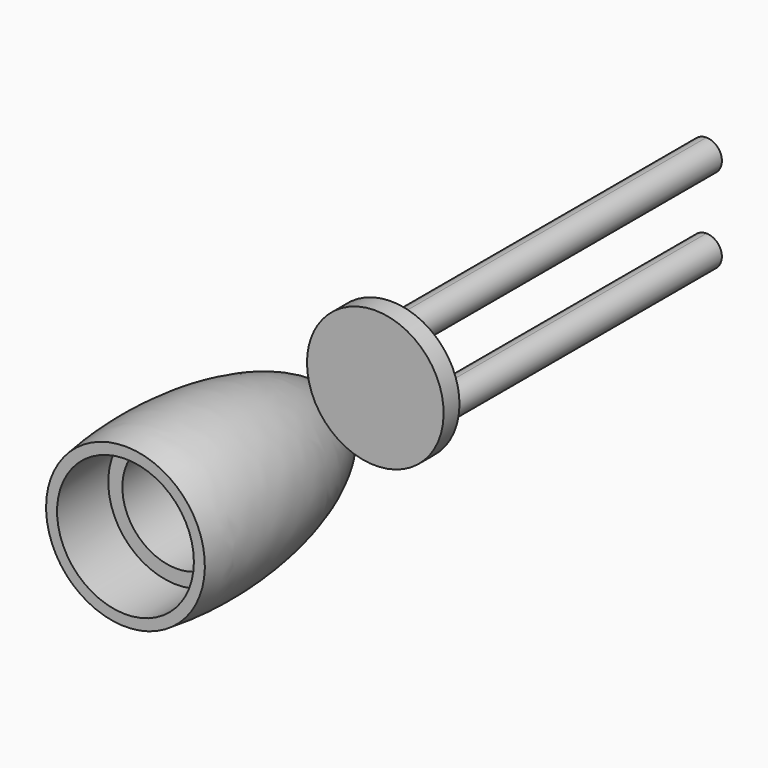
from build123d import *

# Parameters (mm, degrees)
F3_DEPTH  = 50.8
F5_DEPTH  = 25.4
F6_R      = 6.9659499211
F7_DEPTH  = 17.78
F9_DEPTH  = 2.54
F11_DEPTH = 50.8
F13_ANGLE = 180


# Not quite as in the source:
# - a feature of the source that left no trace in its solid (it failed there, or was rolled back) is left out


with BuildPart() as f1:
    # F0 (on Top) → F1 (revolve)
    with BuildSketch(Plane.XY):
        with BuildLine():
            Line((0, -25.4172701389), (0, 25.4172701389))
            add(Edge.make_bspline(
                [(0, 25.4172701389), (-10.7599851836, 25.4172701389), (-10.7599851836, 0), (-10.7599851836, -25.4172701389), (0, -25.4172701389)],
                knots=[0, 0, 0, 1.5707963268, 1.5707963268, 3.1415926536, 3.1415926536, 3.1415926536], degree=2, weights=[1, 0.7071067812, 1, 0.7071067812, 1]))
        make_face()
    revolve(axis=Axis((0, 0, 0), (0, -1, 0)))

    # F2 (on Top) → F3 (cut, symmetric)
    with BuildSketch(Plane.XY):
        Polygon((-21.9557732344, -8.2086902112), (-21.9557732344, -29.9666617066), (26.3073667884, -29.9666617066), (26.3073667884, -8.2086902112), (0, -8.2086902112), align=None)
    extrude(amount=F3_DEPTH, both=True, mode=Mode.SUBTRACT)

    # F4 (on Front) → F5 (cut)
    with BuildSketch(Plane.XZ):
        with BuildLine():
            ThreePointArc((6.4771380141, 5.9206375121), (-8.1806662987, -3.1755258324), (8.7753783624, 0))
            ThreePointArc((8.7753783624, 0), (8.1806662987, 3.1755258324), (6.4771380141, 5.9206375121))
        make_face()
    extrude(amount=F5_DEPTH, mode=Mode.SUBTRACT)

    # F6 (on Front) → F7 (cut)
    with BuildSketch(Plane.XZ):
        Circle(F6_R)
    extrude(amount=-F7_DEPTH, mode=Mode.SUBTRACT)


with BuildPart() as f9:
    # F8 (on Front) → F9 (new body)
    with BuildSketch(Plane.XZ):
        with BuildLine():
            ThreePointArc((-24.6360594414, 31.8792475073), (-40.4608681572, 24.7604353594), (-23.2805613394, 27.1974653006))
            ThreePointArc((-23.2805613394, 27.1974653006), (-23.6262545215, 29.6344952417), (-24.6360594414, 31.8792475073))
        make_face()
    extrude(amount=F9_DEPTH)

    # F10 (on face) → F11 (join)
    with BuildSketch(Plane.XZ.offset(2.54)):
        with BuildLine():
            Line((-31.8433828021, 31.7468605936), (-31.8433828021, 33.7344894722))
            ThreePointArc((-31.8433828021, 33.7344894722), (-33.8310116807, 31.7468605936), (-31.8433828021, 29.759231715))
            Line((-31.8433828021, 29.759231715), (-31.8433828021, 31.7468605936))
        make_face()
        with BuildLine():
            ThreePointArc((-29.8557539234, 31.7468605936), (-30.4379169435, 33.1523264521), (-31.8433828021, 33.7344894722))
            Line((-31.8433828021, 33.7344894722), (-31.8433828021, 31.7468605936))
            Line((-31.8433828021, 31.7468605936), (-29.8557539234, 31.7468605936))
        make_face()
        with BuildLine():
            Line((-29.8557539234, 31.7468605936), (-31.8433828021, 31.7468605936))
            Line((-31.8433828021, 31.7468605936), (-31.8433828021, 29.759231715))
            ThreePointArc((-31.8433828021, 29.759231715), (-30.4379169435, 30.341394735), (-29.8557539234, 31.7468605936))
        make_face()
        with BuildLine():
            ThreePointArc((-31.8433828021, 22.9071260446), (-33.8245828021, 20.9259260446), (-31.8433828021, 18.9447260446))
            Line((-31.8433828021, 18.9447260446), (-31.8433828021, 20.9259260446))
            Line((-31.8433828021, 20.9259260446), (-31.8433828021, 22.9071260446))
        make_face()
        with BuildLine():
            ThreePointArc((-29.8694822943, 21.0958384504), (-30.5038823389, 22.3856835413), (-31.8433828021, 22.9071260446))
            Line((-31.8433828021, 22.9071260446), (-31.8433828021, 20.9259260446))
            Line((-31.8433828021, 20.9259260446), (-29.8694822943, 21.0958384504))
        make_face()
        with BuildLine():
            Line((-31.8433828021, 20.9259260446), (-31.8433828021, 18.9447260446))
            ThreePointArc((-31.8433828021, 18.9447260446), (-30.4424628472, 19.5250060897), (-29.8621828021, 20.9259260446))
            ThreePointArc((-29.8621828021, 20.9259260446), (-29.8640085163, 21.0109606085), (-29.8694822943, 21.0958384504))
            Line((-29.8694822943, 21.0958384504), (-31.8433828021, 20.9259260446))
        make_face()
    extrude(amount=F11_DEPTH)


with BuildPart() as f9_1:
    # F13: moved
    add(f9.part.rotate(Axis((0, 0, 27.2469166666), (0, 0, -1)), F13_ANGLE))


with BuildPart() as f1_1:
    # F14: moved
    add(f1.part.moved(Location((0, 8.2042, 0))))


solid = Compound([f9_1.part, f1_1.part])
